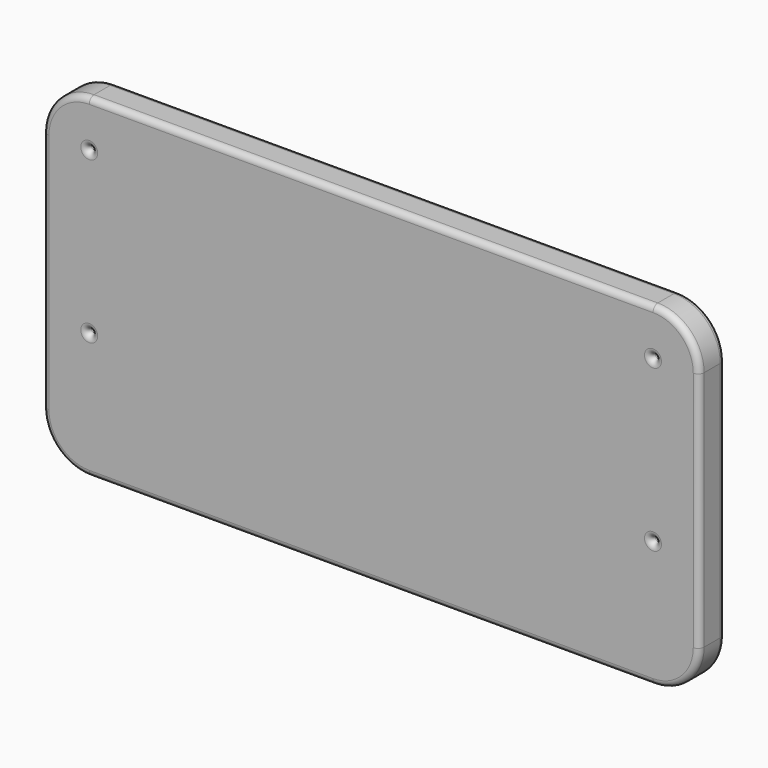
from build123d import *

# Parameters (mm, degrees)
F0_R     = 1.524
F1_DEPTH = 10.16
F2_R     = 3.81
F3_R     = 3.81


# Not quite as in the source:
# - a feature names something its author has since deleted; it is built from what else it names


with BuildPart() as f1:
    # F0 (on Front) → F1 (new body, symmetric)
    with BuildSketch(Plane.XZ):
        with BuildLine():
            Line((16.592341423, -245.2794238949), (-339.007658577, -245.2794238949))
            ThreePointArc((-339.007658577, -245.2794238949), (-359.6622476554, -253.8348348164), (-368.217658577, -274.4894238949))
            Line((-368.217658577, -274.4894238949), (-368.217658577, -426.8894238949))
            ThreePointArc((-368.217658577, -426.8894238949), (-359.6622476554, -447.5440129733), (-339.007658577, -456.0994238949))
            Line((-339.007658577, -456.0994238949), (16.592341423, -456.0994238949))
            ThreePointArc((16.592341423, -456.0994238949), (37.2469305015, -447.5440129733), (45.802341423, -426.8894238949))
            Line((45.802341423, -426.8894238949), (45.802341423, -274.4894238949))
            ThreePointArc((45.802341423, -274.4894238949), (37.2469305015, -253.8348348164), (16.592341423, -245.2794238949))
        make_face()
        with Locations((-339.007658577, -376.0894238949)):
            Circle(F0_R, mode=Mode.SUBTRACT)
        with Locations((16.592341423, -376.0894238949)):
            Circle(F0_R, mode=Mode.SUBTRACT)
        with Locations((-339.007658577, -274.4894238949)):
            Circle(F0_R, mode=Mode.SUBTRACT)
        with Locations((16.592341423, -274.4894238949)):
            Circle(F0_R, mode=Mode.SUBTRACT)
    extrude(amount=F1_DEPTH, both=True)

    # F2
    f2_edges = [f1.edges().sort_by_distance(p)[0] for p in [
        (45.802341, -10.16, -350.689424),
        (37.246931, -10.16, -253.834835),
        (-161.207659, -10.16, -245.279424),
        (-359.662248, -10.16, -253.834835),
        (-368.217659, -10.16, -350.689424),
        (-359.662248, -10.16, -447.544013),
        (-161.207659, -10.16, -456.099424),
        (37.246931, -10.16, -447.544013),
        (-340.531659, -10.16, -376.089424),
        (15.068341, -10.16, -376.089424),
        (-340.531659, -10.16, -274.489424),
        (15.068341, -10.16, -274.489424),
    ]]
    fillet(f2_edges, radius=F2_R)

    # F3
    f3_edges = [f1.edges().sort_by_distance(p)[0] for p in [
        (45.802341, 10.16, -350.689424),
        (37.246931, 10.16, -253.834835),
        (-161.207659, 10.16, -245.279424),
        (-359.662248, 10.16, -253.834835),
        (-368.217659, 10.16, -350.689424),
        (-359.662248, 10.16, -447.544013),
        (-161.207659, 10.16, -456.099424),
        (37.246931, 10.16, -447.544013),
        (-340.531659, 10.16, -376.089424),
        (15.068341, 10.16, -376.089424),
        (-340.531659, 10.16, -274.489424),
        (15.068341, 10.16, -274.489424),
        (-367.101735, -9.044077, -426.889424),
        (-359.662248, -6.35, -447.544013),
        (-356.968171, -10.16, -444.849936),
        (-339.007659, -9.044077, -454.983501),
    ]]
    fillet(f3_edges, radius=F3_R)


solid = f1.part
